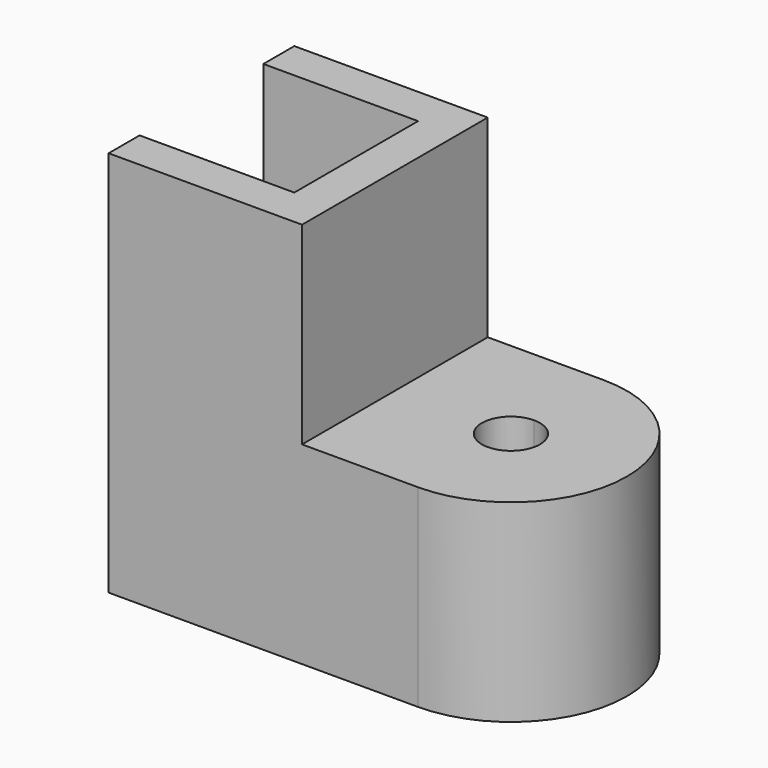
from build123d import *

# Parameters (mm, degrees)
F1_DEPTH  = 20
F2_START  = 10
F1_FACE_R = 1.5
F2_DEPTH  = 10


# Not quite as in the source:
# - a feature names something its author has since deleted; it is built from what else it names


with BuildPart() as f1:
    # F0 (on Top) → F1 (new body)
    with BuildSketch(Plane.XY):
        Polygon((8, 0), (0, 0), (0, -2), (10, -2), (10, 4), (10, 10), (0, 10), (0, 8), (8, 8), align=None)
        with BuildLine():
            Line((16, 2.5), (16, -2))
            ThreePointArc((16, -2), (22, 4), (16, 10))
            Line((16, 10), (16, 5.5))
            ThreePointArc((16, 5.5), (17.0606601718, 5.0606601718), (17.5, 4))
            ThreePointArc((17.5, 4), (17.0606601718, 2.9393398282), (16, 2.5))
        make_face()
        with BuildLine():
            ThreePointArc((10, 4), (11.7573593129, -0.2426406871), (16, -2))
            Line((16, -2), (16, 2.5))
            ThreePointArc((16, 2.5), (14.5, 4), (16, 5.5))
            Line((16, 5.5), (16, 10))
            ThreePointArc((16, 10), (11.7573593129, 8.2426406871), (10, 4))
        make_face()
        with BuildLine():
            Line((16, 10), (10, 10))
            Line((10, 10), (10, 4))
            ThreePointArc((10, 4), (11.7573593129, 8.2426406871), (16, 10))
        make_face()
        with BuildLine():
            Line((10, 4), (10, -2))
            Line((10, -2), (16, -2))
            ThreePointArc((16, -2), (11.7573593129, -0.2426406871), (10, 4))
        make_face()
    extrude(amount=F1_DEPTH)

    # F0 (on Top) + F1_face (on face) → F2 (cut)
    with BuildSketch(Plane.XY.offset(F2_START)):
        with BuildLine():
            Line((16, 2.5), (16, -2))
            ThreePointArc((16, -2), (22, 4), (16, 10))
            Line((16, 10), (16, 5.5))
            ThreePointArc((16, 5.5), (17.0606601718, 5.0606601718), (17.5, 4))
            ThreePointArc((17.5, 4), (17.0606601718, 2.9393398282), (16, 2.5))
        make_face()
        with BuildLine():
            ThreePointArc((10, 4), (11.7573593129, -0.2426406871), (16, -2))
            Line((16, -2), (16, 2.5))
            ThreePointArc((16, 2.5), (14.5, 4), (16, 5.5))
            Line((16, 5.5), (16, 10))
            ThreePointArc((16, 10), (11.7573593129, 8.2426406871), (10, 4))
        make_face()
        with BuildLine():
            Line((10, 4), (10, -2))
            Line((10, -2), (16, -2))
            ThreePointArc((16, -2), (11.7573593129, -0.2426406871), (10, 4))
        make_face()
        with BuildLine():
            Line((16, 10), (10, 10))
            Line((10, 10), (10, 4))
            ThreePointArc((10, 4), (11.7573593129, 8.2426406871), (16, 10))
        make_face()
    with BuildSketch(Plane(origin=(12.4841125556, 4, 20), x_dir=(1, 0, 0), z_dir=(0, 0, 1)).offset(F2_START)):
        with BuildLine():
            Line((-4.4841125556, -4), (-12.4841125556, -4))
            Line((-12.4841125556, -4), (-12.4841125556, -6))
            Line((-12.4841125556, -6), (3.5158874444, -6))
            ThreePointArc((3.5158874444, -6), (9.5158874444, 0), (3.5158874444, 6))
            Line((3.5158874444, 6), (-12.4841125556, 6))
            Line((-12.4841125556, 6), (-12.4841125556, 4))
            Line((-12.4841125556, 4), (-4.4841125556, 4))
            Line((-4.4841125556, 4), (-4.4841125556, -4))
        make_face()
        with Locations((3.5158874444, 0)):
            Circle(F1_FACE_R, mode=Mode.SUBTRACT)
    extrude(amount=F2_DEPTH, mode=Mode.SUBTRACT)


solid = f1.part
